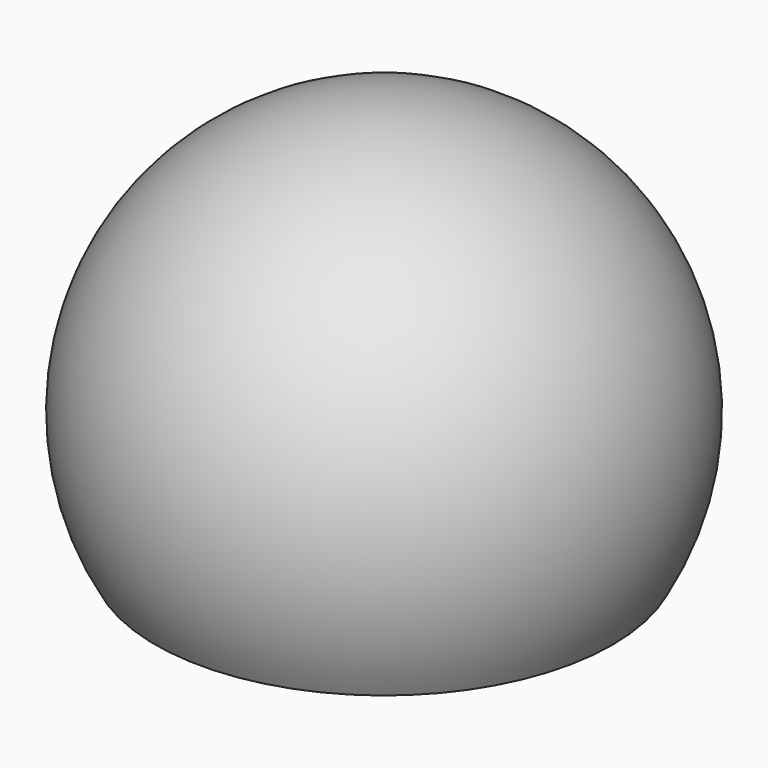
from build123d import *

# Parameters (mm, degrees)
F2_R = 1.19999
F3_R = 1.5


# Not quite as in the source:
# - a fillet or chamfer is up to 0.001 mm smaller than in the source, because OpenCascade refuses the exact size


with BuildPart() as f1:
    # F0 (on Front) → F1 (revolve)
    with BuildSketch(Plane.XZ):
        with BuildLine():
            Line((0, 22.8), (0, 24))
            ThreePointArc((0, 24), (-13.8564064606, 16), (-13.8564064606, 0))
            Line((-13.8564064606, 0), (-12.451505933, 0))
            ThreePointArc((-12.451505933, 0), (-13.8946821516, 13.0968429353), (-4.325, 22.1539526282))
            ThreePointArc((-4.325, 22.1539526282), (-3.7282728081, 22.322708608), (-3.125, 22.4663186402))
            ThreePointArc((-3.125, 22.4663186402), (-1.571382214, 22.7163432257), (0, 22.8))
        make_face()
        with BuildLine():
            Line((-3.125, 17.9663186402), (-3.125, 22.4663186402))
            ThreePointArc((-3.125, 22.4663186402), (-3.7282728081, 22.322708608), (-4.325, 22.1539526282))
            Line((-4.325, 22.1539526282), (-4.325, 17.9663186402))
            Line((-4.325, 17.9663186402), (-3.125, 17.9663186402))
        make_face()
    revolve(axis=Axis((0, 0, 23.4), (0, 0, 1)))

    # F2 (radius 1.2 in the source; OpenCascade refuses exactly that, so slightly less here)
    f2_edges = [f1.edges().sort_by_distance(p)[0] for p in [
        (3.125, 0, 17.966319),
    ]]
    fillet(f2_edges, radius=F2_R)

    # F3
    f3_edges = [f1.edges().sort_by_distance(p)[0] for p in [
        (4.325, 0, 22.153953),
    ]]
    fillet(f3_edges, radius=F3_R)


solid = f1.part
